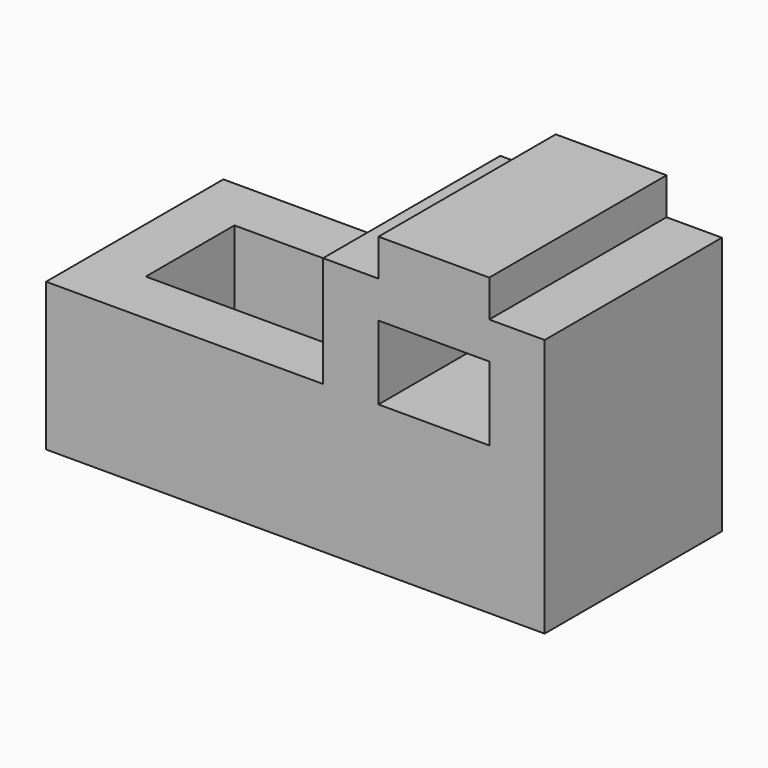
from build123d import *

# Parameters (mm, degrees)
F0_W      = 2743.2
F0_H      = 1625.6
F1_DEPTH  = 1219.2
F2_W      = 304.8
F2_H      = 203.2
F3_DEPTH  = 1219.201
F5_DEPTH  = 1219.201
F9_W      = 609.6
F9_H      = 406.4
F10_DEPTH = 1219.201
F11_W     = 1219.2
F11_H     = 609.6
F12_DEPTH = 812.801


# Not quite as in the source:
# - a feature of the source that left no trace in its solid (it failed there, or was rolled back) is left out
# - a pattern or mirror of a feature is missing from the dataset's text; its kind, count and spacing are read off the source's solid


with BuildPart() as f1:
    # F0 (on Front) → F1 (new body)
    with BuildSketch(Plane.XZ):
        with Locations((-1318.6722079277, 774.8354399085)):
            Rectangle(F0_W, F0_H)
    extrude(amount=F1_DEPTH)

    # F2 (on face) → F3 (cut, through all)
    with BuildSketch(Plane.XZ.offset(1219.2)):
        with Locations((-99.4722079277, 1486.0354399085)):
            Rectangle(F2_W, F2_H)
    f3 = extrude(amount=-F3_DEPTH, mode=Mode.SUBTRACT)

    # F3_copies: F3 across plane
    add(f3.mirror(Plane(origin=(-556.672208, 0, 0), x_dir=(0, 0, -1), z_dir=(-1, 0, 0))), mode=Mode.SUBTRACT)

    # F4 (on face) → F5 (cut, through all)
    with BuildSketch(Plane.XZ.offset(1219.2)):
        Polygon((-1166.2722079277, 1587.6354399085), (-2690.2722079277, 1587.6354399085), (-2690.2722079277, 774.8354399085), (-1166.2722079277, 774.8354399085), (-1166.2722079277, 1384.4354399085), align=None)
    extrude(amount=-F5_DEPTH, mode=Mode.SUBTRACT)

    # F9 (on face) → F10 (cut, through all)
    with BuildSketch(Plane.XZ.offset(1219.2)):
        with Locations((-556.6722079277, 978.0354399085)):
            Rectangle(F9_W, F9_H)
    extrude(amount=-F10_DEPTH, mode=Mode.SUBTRACT)

    # F11 (on face) → F12 (cut, through all)
    with BuildSketch(Plane.XY.offset(774.8354399085)):
        with Locations((-1775.8722079277, -609.6)):
            Rectangle(F11_W, F11_H)
    extrude(amount=-F12_DEPTH, mode=Mode.SUBTRACT)


solid = f1.part
